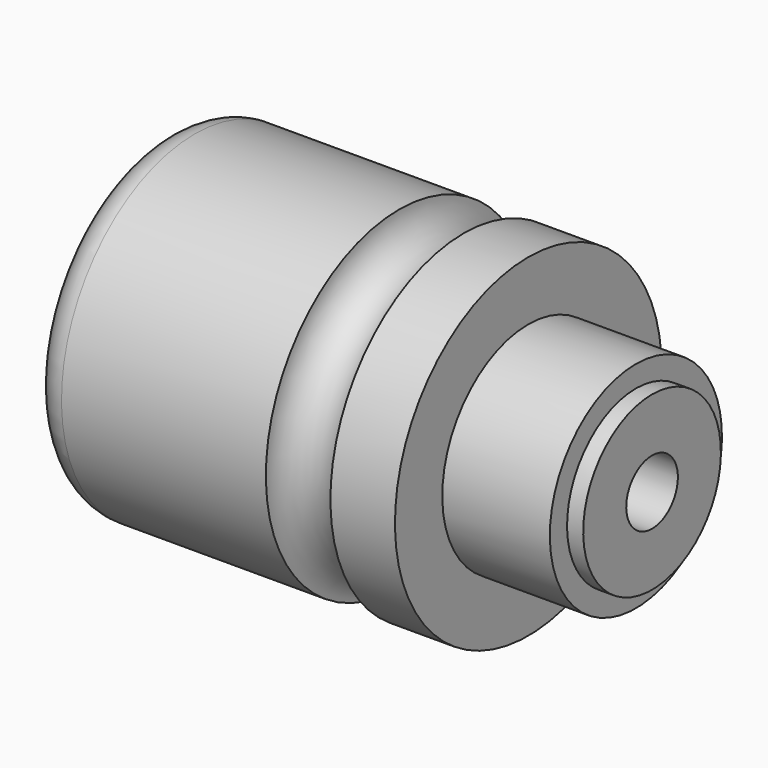
from build123d import *

# Parameters (mm, degrees)
F4_R = 5.99999


# Not quite as in the source:
# - a fillet or chamfer is up to 0.001 mm smaller than in the source, because OpenCascade refuses the exact size


with BuildPart() as f1:
    # F0 (on Front) → F1 (revolve)
    with BuildSketch(Plane.XZ):
        with BuildLine():
            Line((-7.4487626523, 0), (0, 0))
            Line((0, 0), (83.5512373477, 0))
            Line((83.5512373477, 0), (83.5512373477, 16))
            Line((83.5512373477, 16), (80.5512373477, 16))
            Line((80.5512373477, 16), (80.5512373477, 20))
            Line((80.5512373477, 20), (60.5512373477, 20))
            Line((60.5512373477, 20), (60.5512373477, 31))
            Line((60.5512373477, 31), (48.5512373477, 31))
            ThreePointArc((48.5512373477, 31), (42.5512373477, 25), (36.5512373477, 31))
            Line((36.5512373477, 31), (-7.4487626523, 31))
            Line((-7.4487626523, 31), (-7.4487626523, 0))
        make_face()
    revolve(axis=Axis((38.0512373477, 0, 0), (1, 0, 0)))

    # F2 (on Front) → F3 (revolve, cut)
    with BuildSketch(Plane.XZ):
        Polygon((-8.5385272913, 25), (-8.5385272913, 0), (90.8953762729, 0), (90.8953762729, 6), (23.9614727087, 6), (23.9614727087, 16), (15.9614727087, 16), (15.9614727087, 20), (8.9614727087, 20), (8.9614727087, 12.5), (5.9614727087, 12.5), (5.9614727087, 16), (-6.0385272913, 16), (-6.0385272913, 25), align=None)
    revolve(axis=Axis((41.1784244908, 0, 0), (-1, 0, 0)), mode=Mode.SUBTRACT)

    # F4 (radius 6 in the source; OpenCascade refuses exactly that, so slightly less here)
    f4_edges = [f1.edges().sort_by_distance(p)[0] for p in [
        (-7.448763, 0, -31),
    ]]
    fillet(f4_edges, radius=F4_R)


solid = f1.part
